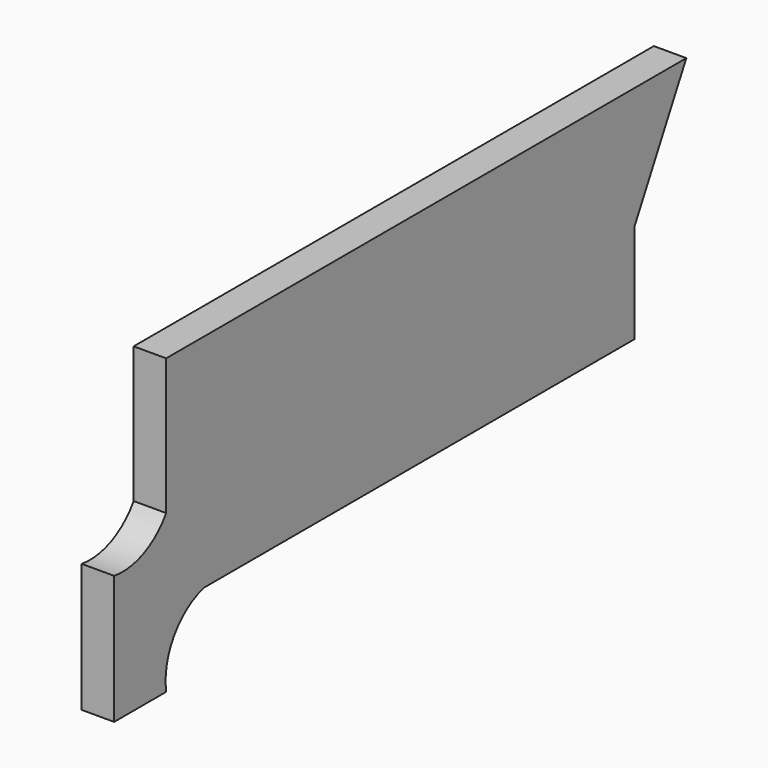
from build123d import *

# Parameters (mm, degrees)
F1_DEPTH = 6.35


# Not quite as in the source:
# - a feature names something its author has since deleted; it is built from what else it names


with BuildPart() as f1:
    # F0 (on Right) → F1 (new body)
    with BuildSketch(Plane.YZ):
        with BuildLine():
            Line((10.1997445822, -25.9578457783), (10.1997445822, -51.0764221646))
            Line((10.1997445822, -51.0764221646), (22.8997445822, -51.0764221646))
            ThreePointArc((22.8997445822, -51.0764221646), (24.7978912955, -42.2422146629), (32.0898325185, -36.9061321742))
            Line((32.0898325185, -36.9061321742), (137.1997445822, -36.9061321742))
            Line((137.1997445822, -36.9061321742), (137.2000693373, -17.6021321769))
            Line((137.2000693373, -17.6021321769), (149.8997445822, 6.2824831575))
            Line((149.8997445822, 6.2824831575), (137.1997445822, 6.2824831575))
            Line((137.1997445822, 6.2824831575), (22.8997445822, 6.2824831575))
            Line((22.8997445822, 6.2824831575), (22.8997445822, -20.3278172679))
            ThreePointArc((22.8997445822, -20.3278172679), (17.3877746683, -25.0332272954), (10.1997445822, -25.9578457783))
        make_face()
    extrude(amount=F1_DEPTH)


solid = f1.part
